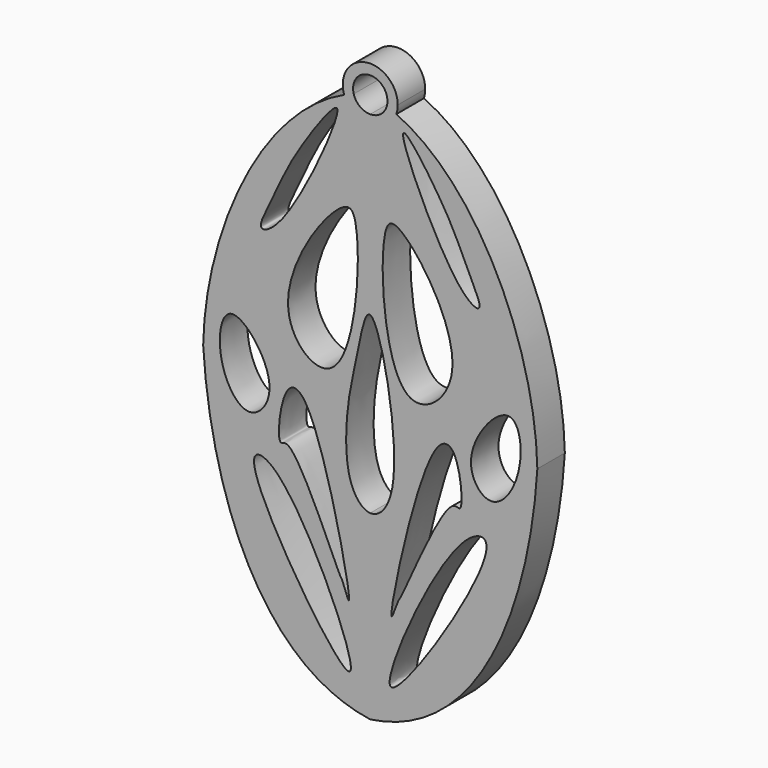
from build123d import *

# Parameters (mm, degrees)
F1_DEPTH = 2.5


with BuildPart() as f1:
    # F0 (on Front) → F1 (new body)
    with BuildSketch(Plane.XZ):
        with BuildLine():
            ThreePointArc((1.9001480208, 19.3759507221), (1.9748792421, 19.6840063603), (2, 19.9999999982))
            ThreePointArc((2, 19.9999999982), (0, 21.9999999982), (-2, 19.9999999982))
            ThreePointArc((-2, 19.9999999982), (-1.9748792421, 19.6840063603), (-1.9001480208, 19.3759507221))
            add(Edge.make_bspline(
                [(-1.202520158, 19.6587592186), (-1.4378422898, 19.5740568966), (-1.6704207632, 19.4796395721), (-1.9001480208, 19.3759507221)],
                knots=[1.3489510655, 1.3489510655, 1.3489510655, 1.3489510655, 2.1559793392, 2.1559793392, 2.1559793392, 2.1559793392], degree=3))
            ThreePointArc((-1.202520158, 19.6587592186), (-0.1722640452, 21.2380731377), (1.25, 19.9999999982))
            ThreePointArc((1.25, 19.9999999982), (1.2380731395, 19.827735953), (1.202520158, 19.6587592186))
            add(Edge.make_bspline(
                [(1.202520158, 19.6587592186), (1.4378422898, 19.5740568966), (1.6704207632, 19.4796395721), (1.9001480208, 19.3759507221)],
                knots=[1.3489510655, 1.3489510655, 1.3489510655, 1.3489510655, 2.1559793392, 2.1559793392, 2.1559793392, 2.1559793392], degree=3))
        make_face()
        with BuildLine():
            add(Edge.make_bspline(
                [(1.9001480208, 19.3759507221), (7.9482510216, 16.646101198), (12.0200971287, 7.4898998172), (12.1529570481, 0)],
                knots=[2.1559793392, 2.1559793392, 2.1559793392, 2.1559793392, 23.4028708696, 23.4028708696, 23.4028708696, 23.4028708696], degree=3))
            ThreePointArc((1.9001480208, 19.3759507221), (1.17300926, 18.3801082499), (0, 17.9999999982))
            ThreePointArc((0, 17.9999999982), (-1.17300926, 18.3801082499), (-1.9001480208, 19.3759507221))
            add(Edge.make_bspline(
                [(-1.9001480208, 19.3759507221), (-7.9482510216, 16.646101198), (-12.0200971287, 7.4898998172), (-12.1529570481, 0)],
                knots=[2.1559793392, 2.1559793392, 2.1559793392, 2.1559793392, 23.4028708696, 23.4028708696, 23.4028708696, 23.4028708696], degree=3))
            add(Edge.make_bspline(
                [(-12.1529570481, 0), (-11.6323980269, -8.6323668898), (-8.229375817, -18.8102871179), (0, -20)],
                knots=[0.4946900023, 0.4946900023, 0.4946900023, 0.4946900023, 1, 1, 1, 1], degree=3))
            add(Edge.make_bspline(
                [(12.1529570481, 0), (11.6323980269, -8.6323668898), (8.229375817, -18.8102871179), (0, -20)],
                knots=[0.4946900023, 0.4946900023, 0.4946900023, 0.4946900023, 1, 1, 1, 1], degree=3))
        make_face()
        with BuildLine():
            add(Edge.make_bspline(
                [(-1.5527566429, -17.4377914518), (-2.507538092, -17.4940520021), (-10.5571136627, -5.2007068229), (-5.6960675536, -5.7349279551), (-0.6338677843, -17.3836458744), (-1.5527566429, -17.4377914518)],
                knots=[0, 0, 0, 0, 0.4313585826, 0.5848572509, 1, 1, 1, 1], degree=3))
        make_face(mode=Mode.SUBTRACT)
        with BuildLine():
            add(Edge.make_bspline(
                [(-10.0579150021, 2.6950780302), (-10.8335012017, 2.6239571095), (-11.3893383856, -0.5754955495), (-8.9369452022, -4.3128803286), (-6.1970362856, -0.8587037773), (-9.1288312743, 2.7802746083), (-10.0579150021, 2.6950780302)],
                knots=[0, 0, 0, 0, 0.239516499, 0.4911309284, 0.7130804005, 1, 1, 1, 1], degree=3))
        make_face(mode=Mode.SUBTRACT)
        with BuildLine():
            add(Edge.make_bspline(
                [(-1.5527566429, -12.8868818283), (-1.629879466, -12.9179285722), (-2.0778528813, -11.5431030884), (-2.1930131483, -11.7709361584), (-5.6169197113, -3.4195948771), (-6.8628530205, -4.9906650673), (-6.4660380574, -0.3570307542), (-3.8338646652, -0.4953668458), (-1.3130294956, -12.7903767078), (-1.5527566429, -12.8868818283)],
                knots=[0, 0, 0, 0, 0.0953626996, 0.1435392696, 0.3852400388, 0.4464543252, 0.6047860806, 0.7035763602, 1, 1, 1, 1], degree=3))
        make_face(mode=Mode.SUBTRACT)
        with BuildLine():
            add(Edge.make_bspline(
                [(1.5527566429, -17.4377914518), (2.507538092, -17.4940520021), (10.5571136627, -5.2007068229), (5.6960675536, -5.7349279551), (0.6338677843, -17.3836458744), (1.5527566429, -17.4377914518)],
                knots=[0, 0, 0, 0, 0.4313585826, 0.5848572509, 1, 1, 1, 1], degree=3))
        make_face(mode=Mode.SUBTRACT)
        with BuildLine():
            add(Edge.make_bspline(
                [(1.5527566429, -12.8868818283), (1.629879466, -12.9179285722), (2.0778528813, -11.5431030884), (2.1930131483, -11.7709361584), (5.6169197113, -3.4195948771), (6.8628530205, -4.9906650673), (6.4660380574, -0.3570307542), (3.8338646652, -0.4953668458), (1.3130294956, -12.7903767078), (1.5527566429, -12.8868818283)],
                knots=[0, 0, 0, 0, 0.0953626996, 0.1435392696, 0.3852400388, 0.4464543252, 0.6047860806, 0.7035763602, 1, 1, 1, 1], degree=3))
        make_face(mode=Mode.SUBTRACT)
        with BuildLine():
            add(Edge.make_bspline(
                [(0, -6.7852260545), (0.6819859157, -6.823648977), (2.7953232493, -4.6244677377), (0.77067262, 5.5796490518), (0, 5.8970530517)],
                knots=[0.5942064363, 0.5942064363, 0.5942064363, 0.5942064363, 0.7358484055, 1, 1, 1, 1], degree=3))
            add(Edge.make_bspline(
                [(0, 5.8970530517), (-0.3861457229, 6.056088411), (-0.9442319679, 2.8503765697), (-1.7633874334, -0.2535547354), (-1.8963861077, -5.2807895735), (-0.5612516861, -6.7536052695), (0, -6.7852260545)],
                knots=[0, 0, 0, 0, 0.1323532273, 0.2969409084, 0.4776398149, 0.5942064363, 0.5942064363, 0.5942064363, 0.5942064363], degree=3))
        make_face(mode=Mode.SUBTRACT)
        with BuildLine():
            add(Edge.make_bspline(
                [(10.8954617152, 2e-10), (10.8811011309, -0.1163821385), (10.6328819389, -1.7283159166), (8.9369452022, -4.3128803286), (6.1970362856, -0.8587037773), (9.1288312743, 2.7802746083), (10.0579150021, 2.6950780302)],
                knots=[0.2199542347, 0.2199542347, 0.2199542347, 0.2199542347, 0.239516499, 0.4911309284, 0.7130804005, 1, 1, 1, 1], degree=3))
            add(Edge.make_bspline(
                [(10.0579150021, 2.6950780302), (10.7701559947, 2.6297658377), (11.0569292875, 1.3085777741), (10.8954617152, 2e-10)],
                knots=[0, 0, 0, 0, 0.2199542347, 0.2199542347, 0.2199542347, 0.2199542347], degree=3))
        make_face(mode=Mode.SUBTRACT)
        with BuildLine():
            add(Edge.make_bspline(
                [(-1.9597173668, 12.167849578), (-3.2671084858, 11.4701196865), (-8.3238185403, 4.3836297337), (-1.2171543721, -1.4524826127), (-0.4839324206, 11.6923173391), (-1.5111263135, 12.4072541314), (-1.9597173668, 12.167849578)],
                knots=[0, 0, 0, 0, 0.3226566431, 0.5437780707, 0.8892902963, 1, 1, 1, 1], degree=3))
        make_face(mode=Mode.SUBTRACT)
        with BuildLine():
            add(Edge.make_bspline(
                [(-2.4161490146, 18.3310989374), (-2.6554951791, 18.6351560491), (-6.0172544369, 13.7891634437), (-6.7445339964, 11.6182768527), (-8.5455002356, 8.4084474321), (-5.8578836448, 9.4993259941), (-2.0891260666, 17.9156602641), (-2.4161490146, 18.3310989374)],
                knots=[0, 0, 0, 0, 0.224008914, 0.4105117391, 0.5648440708, 0.6939326118, 1, 1, 1, 1], degree=3))
        make_face(mode=Mode.SUBTRACT)
        with BuildLine():
            add(Edge.make_bspline(
                [(1.9597173668, 12.167849578), (3.2671084858, 11.4701196865), (8.3238185403, 4.3836297337), (1.2171543721, -1.4524826127), (0.4839324206, 11.6923173391), (1.5111263135, 12.4072541314), (1.9597173668, 12.167849578)],
                knots=[0, 0, 0, 0, 0.3226566431, 0.5437780707, 0.8892902963, 1, 1, 1, 1], degree=3))
        make_face(mode=Mode.SUBTRACT)
        with BuildLine():
            add(Edge.make_bspline(
                [(2.4161490146, 18.3310989374), (2.6554951791, 18.6351560491), (6.0172544369, 13.7891634437), (6.7445339964, 11.6182768527), (8.5455002356, 8.4084474321), (5.8578836448, 9.4993259941), (2.0891260666, 17.9156602641), (2.4161490146, 18.3310989374)],
                knots=[0, 0, 0, 0, 0.224008914, 0.4105117391, 0.5648440708, 0.6939326118, 1, 1, 1, 1], degree=3))
        make_face(mode=Mode.SUBTRACT)
        with BuildLine():
            ThreePointArc((0, 17.9999999982), (1.17300926, 18.3801082499), (1.9001480208, 19.3759507221))
            add(Edge.make_bspline(
                [(1.202520158, 19.6587592186), (1.4378422898, 19.5740568966), (1.6704207632, 19.4796395721), (1.9001480208, 19.3759507221)],
                knots=[1.3489510655, 1.3489510655, 1.3489510655, 1.3489510655, 2.1559793392, 2.1559793392, 2.1559793392, 2.1559793392], degree=3))
            ThreePointArc((1.202520158, 19.6587592186), (0.753640838, 19.0027410111), (0, 18.7499999982))
            Line((0, 18.7499999982), (0, 17.9999999982))
        make_face()
        with BuildLine():
            add(Edge.make_bspline(
                [(-1.202520158, 19.6587592186), (-1.4378422898, 19.5740568966), (-1.6704207632, 19.4796395721), (-1.9001480208, 19.3759507221)],
                knots=[1.3489510655, 1.3489510655, 1.3489510655, 1.3489510655, 2.1559793392, 2.1559793392, 2.1559793392, 2.1559793392], degree=3))
            ThreePointArc((-1.9001480208, 19.3759507221), (-1.17300926, 18.3801082499), (0, 17.9999999982))
            Line((0, 17.9999999982), (0, 18.7499999982))
            ThreePointArc((0, 18.7499999982), (-0.753640838, 19.0027410111), (-1.202520158, 19.6587592186))
        make_face()
    extrude(amount=F1_DEPTH)


solid = f1.part
